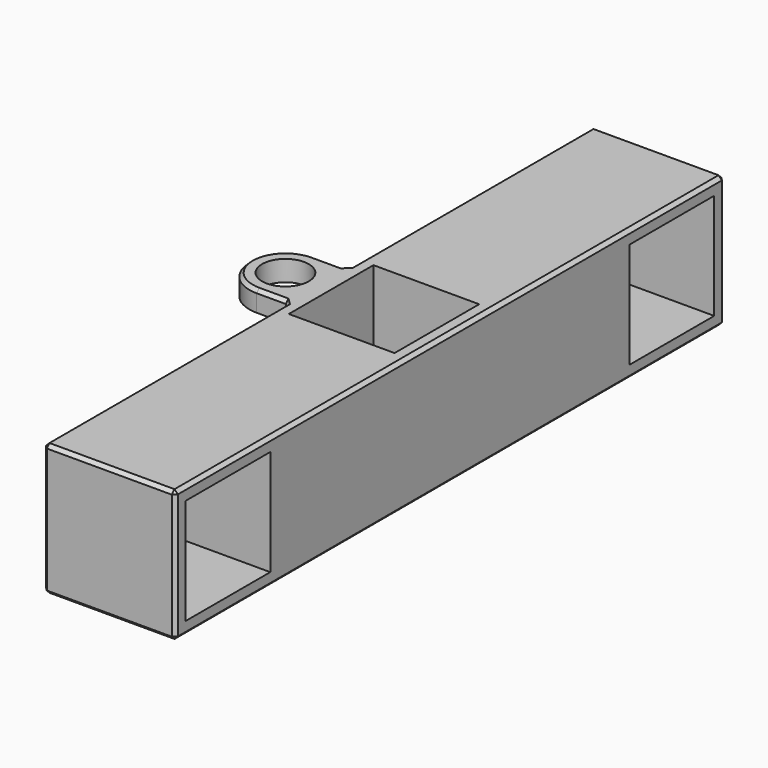
from build123d import *

# Parameters (mm, degrees)
F0_W        = 19.2
F0_H        = 100
F1_DEPTH    = 19.2
F2_W        = 15.4
F2_H        = 15.4
F3_DEPTH    = 18
F4_W        = 20
F4_H        = 10.5
F5_DEPTH    = 3
F6_T1_DEPTH = 29.25
F7_R        = 3.4
F8_DEPTH    = 25
F9_SIZE     = 0.5
F11_W       = 15.4
F11_H       = 15.4
F12_DEPTH   = 18


# Not quite as in the source:
# - a fillet or chamfer that OpenCascade refuses, or shapes differently, is made with other operations: its cross-section is extruded or revolved along the edge and cut away or added
# - a pattern or mirror of a feature is missing from the dataset's text; its kind, count and spacing are read off the source's solid


with BuildPart() as f1:
    # F0 (on Top) → F1 (new body)
    with BuildSketch(Plane.XY):
        Rectangle(F0_W, F0_H)
    extrude(amount=F1_DEPTH)

    # F2 (on face) → F3 (cut)
    with BuildSketch(Plane.YZ.offset(9.6)):
        with Locations((-40.4, 9.6)):
            Rectangle(F2_W, F2_H)
    f3 = extrude(amount=-F3_DEPTH, mode=Mode.SUBTRACT)

    # F3_copies: F3 across plane
    add(f3.mirror(Plane.ZX), mode=Mode.SUBTRACT)

    # F4 (on face) → F5 (join)
    with BuildSketch(Plane.XY.offset(19.2)):
        with Locations((-9.6, 0)):
            Rectangle(F4_W, F4_H)
    extrude(amount=-F5_DEPTH)

    # F6: fillet of radius 5.25 on 2 edges, made by hand

    # F6_s2 → F6_t1 (cut)
    with BuildSketch(Plane.XY.offset(3.075)):
        with BuildLine():
            ThreePointArc((-14.35, 5.25), (-18.0623106012, 3.7123106012), (-19.6, 0))
            Line((-19.6, 0), (-19.6, 5.25))
            Line((-19.6, 5.25), (-14.35, 5.25))
        make_face()
        with BuildLine():
            ThreePointArc((-14.35, -5.25), (-18.0623106012, -3.7123106012), (-19.6, 0))
            Line((-19.6, 0), (-19.6, -5.25))
            Line((-19.6, -5.25), (-14.35, -5.25))
        make_face()
    extrude(amount=F6_T1_DEPTH, mode=Mode.SUBTRACT)

    # F7 (on face) → F8 (cut)
    with BuildSketch(Plane.XY.offset(19.2)):
        with Locations((-14.35, 0)):
            Circle(F7_R)
    extrude(amount=-F8_DEPTH, mode=Mode.SUBTRACT)

    # F9
    f9_edges = [f1.edges().sort_by_distance(p)[0] for p in [
        (-9.6, 0, 0),
        (-9.6, -50, 9.6),
        (-9.6, -27.625, 19.2),
        (-9.6, -5.25, 17.7),
        (-9.6, 0, 16.2),
        (-9.6, 5.25, 17.7),
        (-9.6, 27.625, 19.2),
        (-9.6, 50, 9.6),
        (9.6, -50, 9.6),
        (0, -50, 0),
        (0, -50, 19.2),
        (9.6, 50, 9.6),
        (0, 50, 0),
        (0, 50, 19.2),
        (9.6, 0, 0),
        (9.6, 0, 19.2),
        (-11.975, -5.25, 19.2),
        (-18.062311, -3.712311, 19.2),
        (-18.062311, 3.712311, 19.2),
        (-11.975, 5.25, 19.2),
    ]]
    chamfer(f9_edges, length=F9_SIZE)

    # F11 (on face) → F12 (cut)
    with BuildSketch(Plane.XY.offset(19.2)):
        Rectangle(F11_W, F11_H)
    extrude(amount=-F12_DEPTH, mode=Mode.SUBTRACT)


solid = f1.part
